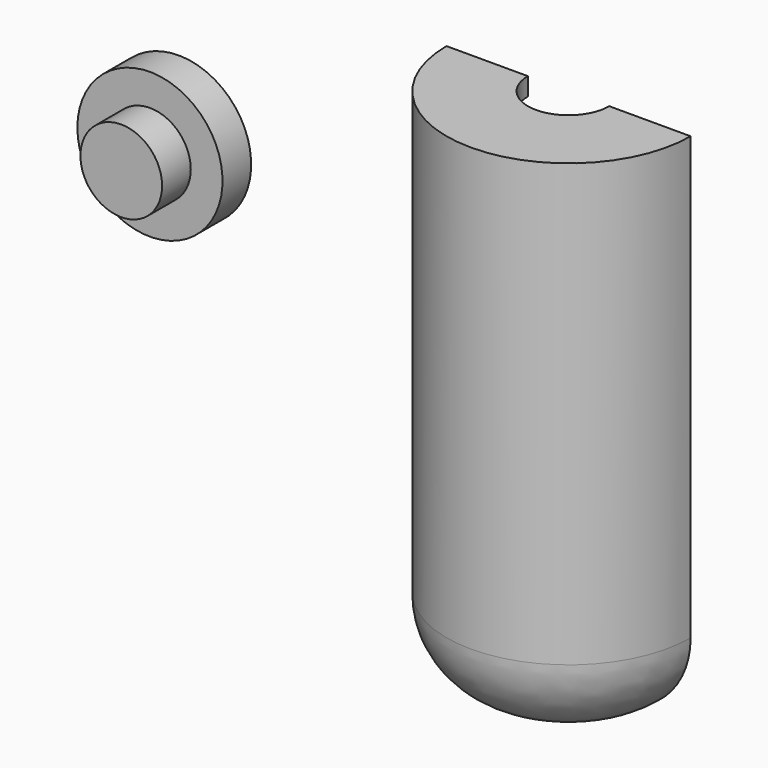
from build123d import *

# Parameters (mm, degrees)
F1_ANGLE = 180
F2_DEPTH = 3
F3_DEPTH = 3
F4_R     = 2.2783423097
F5_DEPTH = 2
F6_R     = 4.0488985141
F6_R_2   = 2.2783423097
F7_DEPTH = 2


with BuildPart() as f1:
    # F0 (on Front) → F1 (revolve)
    with BuildSketch(Plane.XZ):
        with BuildLine():
            Line((11.6213960573, 14.9004508704), (11.6213960573, 0))
            Line((11.6213960573, 0), (8.3194198087, 0))
            Line((8.3194198087, 0), (8.3194198087, -1))
            Line((8.3194198087, -1), (8.3194198087, -5.4323007353))
            Line((8.3194198087, -5.4323007353), (9.3194198087, -5.4323007353))
            ThreePointArc((9.3194198087, -5.4323007353), (11.7051618742, -3.7635274992), (12.6213960573, -1))
            Line((12.6213960573, -1), (12.6213960573, 15.9004508704))
            Line((12.6213960573, 15.9004508704), (12.6213960573, 19.6379758418))
            Line((12.6213960573, 19.6379758418), (12.6213960573, 20.6379758418))
            Line((12.6213960573, 20.6379758418), (8.0798119307, 20.6379758418))
            Line((8.0798119307, 20.6379758418), (8.0798119307, 19.6379758418))
            Line((8.0798119307, 19.6379758418), (11.6213960573, 19.6379758418))
            Line((11.6213960573, 19.6379758418), (11.6213960573, 15.9004508704))
            Line((11.6213960573, 15.9004508704), (9.7232601838, 15.9004508704))
            Line((9.7232601838, 15.9004508704), (7.8655318357, 15.9004508704))
            Line((7.8655318357, 15.9004508704), (7.8655318357, 14.9004508704))
            Line((7.8655318357, 14.9004508704), (9.7232601838, 14.9004508704))
            Line((9.7232601838, 14.9004508704), (11.6213960573, 14.9004508704))
        make_face()
    revolve(axis=Axis((5.8106980287, 0, 17.7692133561), (0, 0, -1)), revolution_arc=F1_ANGLE)

    # F2 (add): a face of the model
    f2_faces = [f1.faces().sort_by_distance(p)[0] for p in [
        (5.8106980287, -3.1312214854, 20.6379758418),
    ]]
    extrude(f2_faces, amount=F2_DEPTH)

    # F3 (cut): a face of the model
    f3_faces = [f1.faces().sort_by_distance(p)[0] for p in [
        (5.8106980287, -2.7365950697, 19.6379758418),
    ]]
    extrude(f3_faces, amount=-F3_DEPTH, mode=Mode.SUBTRACT)


with BuildPart() as f5:
    # F4 (on Front) → F5 (new body)
    with BuildSketch(Plane.XZ):
        with Locations((-17.5498593599, 12.9418279976)):
            Circle(F4_R)
    extrude(amount=F5_DEPTH)

    # F6 (on face) → F7 (join)
    with BuildSketch(Plane(origin=(0, 0, 0), x_dir=(-1, 0, 0), z_dir=(0, 1, 0))):
        with Locations((17.5498593599, 12.9418279976)):
            Circle(F6_R)
        with Locations((17.5498593599, 12.9418279976)):
            Circle(F6_R_2, mode=Mode.SUBTRACT)
        with Locations((17.5498593599, 12.9418279976)):
            Circle(F6_R_2)
    extrude(amount=F7_DEPTH)


solid = Compound([f1.part, f5.part])
